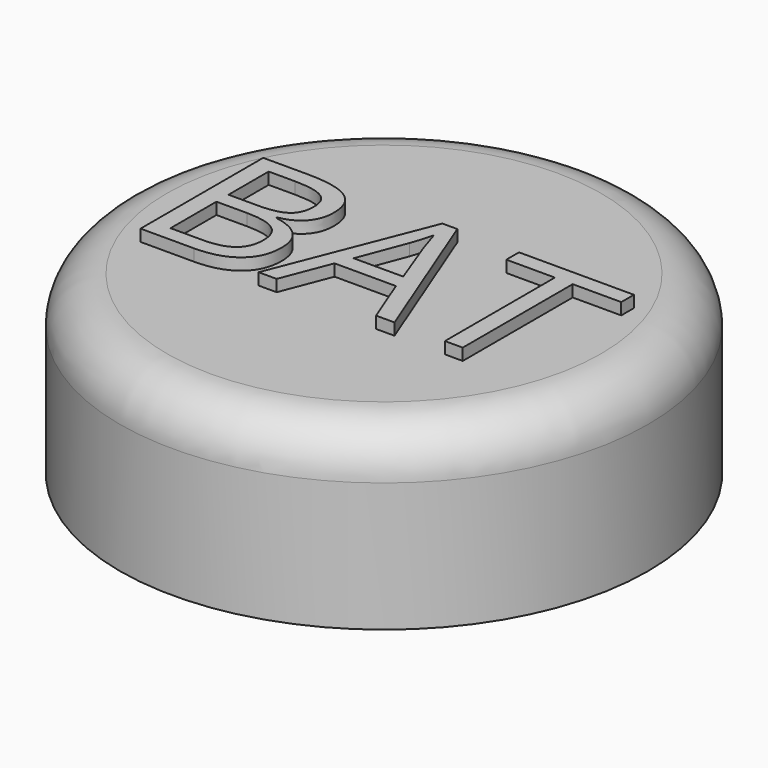
from build123d import *

# Parameters (mm, degrees)
F0_R         = 28.575
F1_DEPTH     = 19.05
F2_R         = 5.08
F3_T         = -2.54
F4_TEXT_SIZE = 23.2303481082
F5_DEPTH     = 1.27
F6_SIZE      = 1.27


# Not quite as in the source:
# - Text() gives the source's letters only with a copy of the font that has no kerning and outlines rounded to 1/6400 em; it was checked with that copy


with BuildPart() as f1:
    # F0 (on Top) → F1 (new body)
    with BuildSketch(Plane.XY):
        Circle(F0_R)
    extrude(amount=F1_DEPTH)

    # F2
    f2_edges = [f1.edges().sort_by_distance(p)[0] for p in [
        (-28.575, 0, 19.05),
    ]]
    fillet(f2_edges, radius=F2_R)

    # F3
    f3_openings = [f1.faces().sort_by_distance(p)[0] for p in [
        (0, 0, 0),
    ]]
    offset(amount=F3_T, openings=f3_openings)

    # F4 (on face) → F5 (join)
    with BuildSketch(Plane.XY.offset(19.05)):
        with Locations((-21.9472343494, -8.3393180164)):
            Text('BAT', F4_TEXT_SIZE, font='Open Sans', text_align=(TextAlign.LEFT, TextAlign.BOTTOM))
    extrude(amount=F5_DEPTH)

    # F6
    f6_edges = [f1.edges().sort_by_distance(p)[0] for p in [
        (-26.035, 0, 0),
    ]]
    chamfer(f6_edges, length=F6_SIZE)


solid = f1.part
